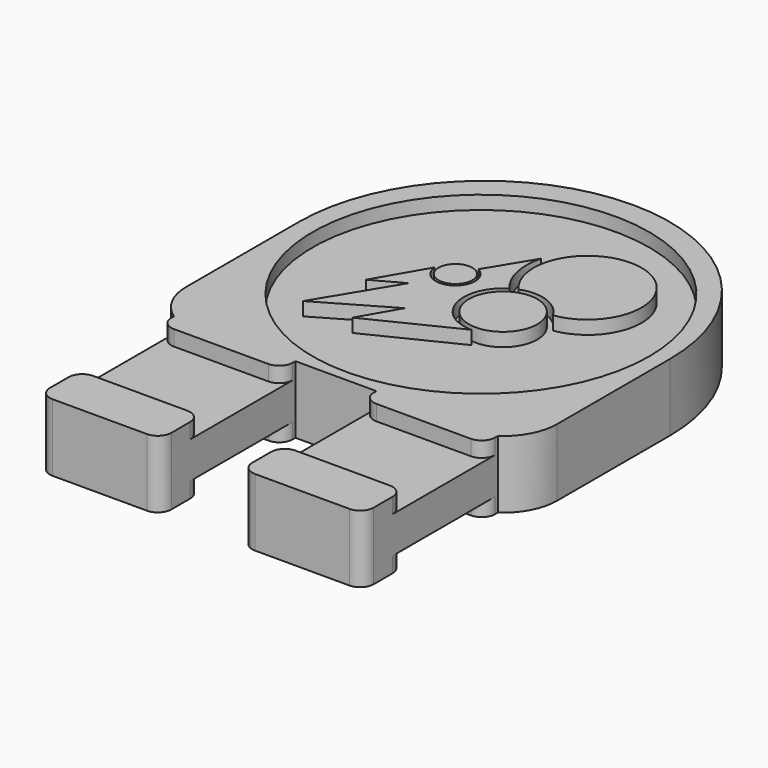
from build123d import *

# Parameters (mm, degrees)
F1_DEPTH    = 3.175
F2_W        = 9.525
F2_H        = 1.4478
F3_DEPTH    = 25.4
F4_R        = 15.842845787
F4_R_2      = 3.2177044056
F4_R_3      = 1.5904309239
F5_DEPTH    = 1.27
F6_T1_DEPTH = 31.75
F6_T3_DEPTH = 27.3506510316
F7_R        = 1.27
F9_DEPTH    = 25.4


# Not quite as in the source:
# - a fillet or chamfer that OpenCascade refuses, or shapes differently, is made with other operations: its cross-section is extruded or revolved along the edge and cut away or added


with BuildPart() as f1:
    # F0 (on Top) → F1 (new body, symmetric)
    with BuildSketch(Plane.XY):
        Polygon((17.7787664203, 21.9838270611), (-17.1462335797, 21.9838270611), (-17.1462335797, -12.9411729389), (-14.9237335797, -12.9411729389), (-14.9237335797, -28.8161729389), (-3.4937335797, -28.8161729389), (-3.4937335797, -12.9411729389), (4.1262664203, -12.9411729389), (4.1262664203, -28.8161729389), (15.5562664203, -28.8161729389), (15.5562664203, -12.9411729389), (17.7787664203, -12.9411729389), align=None)
    extrude(amount=F1_DEPTH, both=True)

    # F2 (on Right) → F3 (cut, symmetric)
    with BuildSketch(Plane.YZ):
        with Locations((-19.2911729389, -2.4511)):
            Rectangle(F2_W, F2_H)
        with Locations((-19.2911729389, 2.4511)):
            Rectangle(F2_W, F2_H)
    extrude(amount=F3_DEPTH, both=True, mode=Mode.SUBTRACT)

    # F4 (on face) → F5 (cut)
    with BuildSketch(Plane.XY.offset(3.175)):
        with Locations((0.4921501707, 3.9010436143)):
            Circle(F4_R)
        with BuildLine():
            Line((-2.1375703251, 6.8868143019), (0.4050256131, 11.0911789057))
            ThreePointArc((0.4050256131, 11.0911789057), (0.3466666466, 8.3599053372), (1.5539010716, 5.9092225511))
            ThreePointArc((1.5539010716, 5.9092225511), (-0.0735190255, 1.7484484648), (3.4811131017, -0.9580488308))
            Line((3.4811131017, -0.9580488308), (-4.5523895124, -4.9100595401))
            Line((-4.5523895124, -4.9100595401), (-2.4823771265, -1.3211422242))
            Line((-2.4823771265, -1.3211422242), (-9.0284545614, -5.1116843583))
            Line((-9.0284545614, -5.1116843583), (-4.7554110557, 1.9540993141))
            Line((-4.7554110557, 1.9540993141), (-7.5469899631, 0.4189560082))
            Line((-7.5469899631, 0.4189560082), (-4.8280507742, 5.1179121089))
            ThreePointArc((-4.8280507742, 5.1179121089), (-1.9693373897, 3.7003874584), (-2.1375703251, 6.8868143019))
        make_face(mode=Mode.SUBTRACT)
        with Locations((3.4971262654, 2.7505044746)):
            Circle(F4_R_2, mode=Mode.SUBTRACT)
        with Locations((-2.9845039712, 5.2444444735)):
            Circle(F4_R_3, mode=Mode.SUBTRACT)
        with BuildLine():
            ThreePointArc((2.1821519983, 6.218135758), (7.6895432258, 14.3852639145), (6.7216994367, 4.5823756229))
            ThreePointArc((6.7216994367, 4.5823756229), (4.7543334077, 6.2394949077), (2.1821519983, 6.218135758))
        make_face(mode=Mode.SUBTRACT)
    extrude(amount=-F5_DEPTH, mode=Mode.SUBTRACT)

    # F6: fillet of radius 5.08 on 4 edges, made by hand

    # F6_s2 → F6_t1 (cut)
    with BuildSketch(Plane.XY.offset(-15.875)):
        with BuildLine():
            ThreePointArc((17.7787664203, 16.9038270611), (16.2908688687, 20.4959295096), (12.6987664203, 21.9838270611))
            Line((12.6987664203, 21.9838270611), (17.7787664203, 21.9838270611))
            Line((17.7787664203, 21.9838270611), (17.7787664203, 16.9038270611))
        make_face()
        with BuildLine():
            ThreePointArc((-12.0662335797, 21.9838270611), (-15.6583360282, 20.4959295096), (-17.1462335797, 16.9038270611))
            Line((-17.1462335797, 16.9038270611), (-17.1462335797, 21.9838270611))
            Line((-17.1462335797, 21.9838270611), (-12.0662335797, 21.9838270611))
        make_face()
    extrude(amount=F6_T1_DEPTH, mode=Mode.SUBTRACT)

    # F6_s4 → F6_t3 (cut)
    with BuildSketch(Plane.XY.offset(-13.6753255158)):
        with BuildLine():
            ThreePointArc((-14.9237335797, -12.9411729388), (-16.5563616403, -11.1169951731), (-17.1462335797, -8.7410427325))
            Line((-17.1462335797, -8.7410427325), (-17.1462335797, -12.9411729389))
            Line((-17.1462335797, -12.9411729389), (-14.9237335797, -12.9411729388))
        make_face()
        with BuildLine():
            ThreePointArc((17.7787664203, -8.7410427325), (17.1888944808, -11.1169951731), (15.5562664203, -12.9411729388))
            Line((15.5562664203, -12.9411729388), (17.7787664203, -12.9411729389))
            Line((17.7787664203, -12.9411729389), (17.7787664203, -8.7410427325))
        make_face()
    extrude(amount=F6_T3_DEPTH, mode=Mode.SUBTRACT)

    # F7
    f7_edges = [f1.edges().sort_by_distance(p)[0] for p in [
        (-14.923734, -14.528673, 2.4511),
        (-3.493734, -14.528673, 2.4511),
        (15.556266, -14.528673, 2.4511),
        (4.126266, -14.528673, 2.4511),
        (15.556266, -14.528673, -2.4511),
        (4.126266, -14.528673, -2.4511),
        (-14.923734, -14.528673, -2.4511),
        (-3.493734, -14.528673, -2.4511),
        (-3.493734, -24.053673, -2.4511),
        (-3.493734, -24.053673, 2.4511),
        (15.556266, -24.053673, -2.4511),
        (15.556266, -24.053673, 2.4511),
        (15.556266, -28.816173, 0),
        (4.126266, -28.816173, 0),
        (-3.493734, -28.816173, 0),
        (-14.923734, -28.816173, 0),
        (-14.923734, -24.053673, 2.4511),
        (-14.923734, -24.053673, -2.4511),
        (4.126266, -24.053673, 2.4511),
        (4.126266, -24.053673, -2.4511),
    ]]
    fillet(f7_edges, radius=F7_R)

    # F8 (on face) → F9 (cut)
    with BuildSketch(Plane.XY.offset(3.175)):
        with BuildLine():
            ThreePointArc((-17.1462335797, 16.9038270611), (-15.6583360282, 20.4959295096), (-12.0662335797, 21.9838270611))
            Line((-12.0662335797, 21.9838270611), (-17.1462335797, 21.9838270611))
            Line((-17.1462335797, 21.9838270611), (-17.1462335797, 16.9038270611))
        make_face()
        with BuildLine():
            ThreePointArc((12.6987664203, 21.9838270611), (16.2908688687, 20.4959295095), (17.7787664203, 16.9038270611))
            Line((17.7787664203, 16.9038270611), (17.7787664203, 21.9838270611))
            Line((17.7787664203, 21.9838270611), (12.6987664203, 21.9838270611))
        make_face()
        with BuildLine():
            ThreePointArc((0.3162664203, 21.9838270611), (12.6641185867, 16.8691792276), (17.7787664203, 4.5213270611))
            Line((17.7787664203, 4.5213270611), (17.7787664203, 16.9038270611))
            ThreePointArc((17.7787664203, 16.9038270611), (16.2908688687, 20.4959295095), (12.6987664203, 21.9838270611))
            Line((12.6987664203, 21.9838270611), (0.3162664203, 21.9838270611))
        make_face()
        with BuildLine():
            ThreePointArc((-17.1462335797, 4.5213270326), (-12.0315857563, 16.8691792175), (0.3162664203, 21.9838270611))
            Line((0.3162664203, 21.9838270611), (-12.0662335797, 21.9838270611))
            ThreePointArc((-12.0662335797, 21.9838270611), (-15.6583360282, 20.4959295096), (-17.1462335797, 16.9038270611))
            Line((-17.1462335797, 16.9038270611), (-17.1462335797, 4.5213270326))
        make_face()
    extrude(amount=-F9_DEPTH, mode=Mode.SUBTRACT)


solid = f1.part
